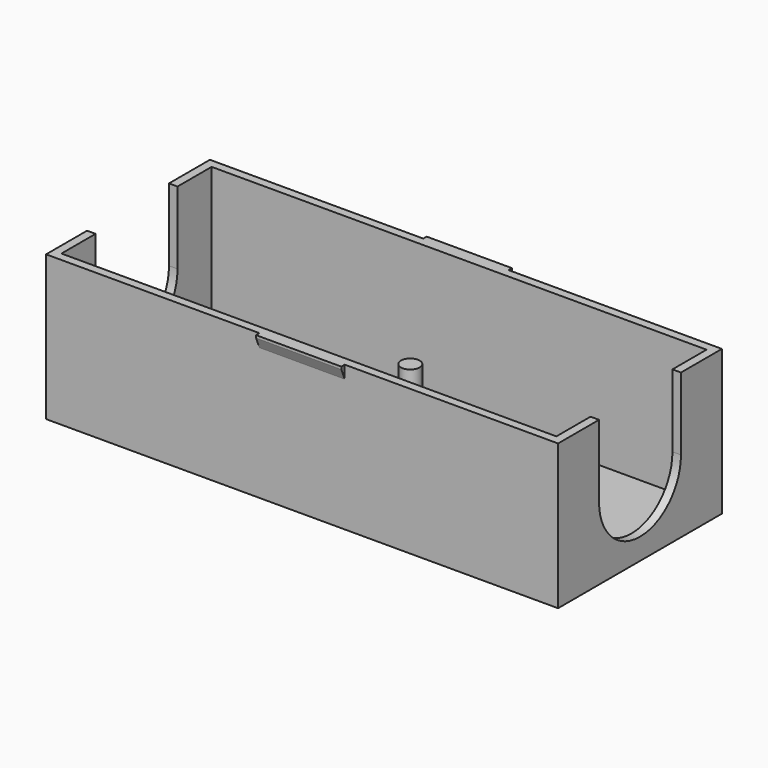
from build123d import *

# Parameters (mm, degrees)
F0_W      = 60
F0_H      = 24
F1_DEPTH  = 17
F2_T      = -1
F3_W      = 10
F3_H      = 1.5
F4_DEPTH  = 0.5
F5_SIZE2  = 1.19999
F5_SIZE   = 0.49999
F8_DEPTH  = 60.001
F9_R      = 1.1
F10_DEPTH = 8


# Not quite as in the source:
# - a fillet or chamfer is up to 0.001 mm smaller than in the source, because OpenCascade refuses the exact size


with BuildPart() as f1:
    # F0 (on Top) → F1 (new body)
    with BuildSketch(Plane.XY):
        Rectangle(F0_W, F0_H)
    extrude(amount=F1_DEPTH)

    # F2
    f2_openings = [f1.faces().sort_by_distance(p)[0] for p in [
        (0, 0, 17),
    ]]
    offset(amount=F2_T, openings=f2_openings)

    # F3 (on face) → F4 (join)
    with BuildSketch(Plane.XZ.offset(12)):
        with Locations((0, 16.25)):
            Rectangle(F3_W, F3_H)
    extrude(amount=F4_DEPTH)

    # F5 (size 0.5 and 1.2 in the source; OpenCascade refuses exactly that, so slightly less here)
    f5_edges = [f1.edges().sort_by_distance(p)[0] for p in [
        (0, -12.5, 15.5),
    ]]
    f5_side = f1.faces().sort_by_distance((0, -12.25, 15.5))[0]
    chamfer(f5_edges, length=F5_SIZE, length2=F5_SIZE2, reference=f5_side)

    # F6: F1 across plane


with BuildPart() as f1_1:
    add(f1.part)
    add(f1.part.mirror(Plane.XZ))

    # F7 (on face) → F8 (cut, through all)
    with BuildSketch(Plane(origin=(-30, 0, 0), x_dir=(0, -1, 0), z_dir=(-1, 0, 0))):
        with BuildLine():
            Line((-6, 17), (-6, 8.5))
            ThreePointArc((-6, 8.5), (0, 2.5), (6, 8.5))
            Line((6, 8.5), (6, 17))
            Line((6, 17), (-6, 17))
        make_face()
    extrude(amount=-F8_DEPTH, mode=Mode.SUBTRACT)

    # F9 (on face) → F10 (join)
    with BuildSketch(Plane.XY.offset(1)):
        with Locations((0, 3.85)):
            Circle(F9_R)
        with Locations((0, -3.85)):
            Circle(F9_R)
    extrude(amount=F10_DEPTH)


solid = f1_1.part
